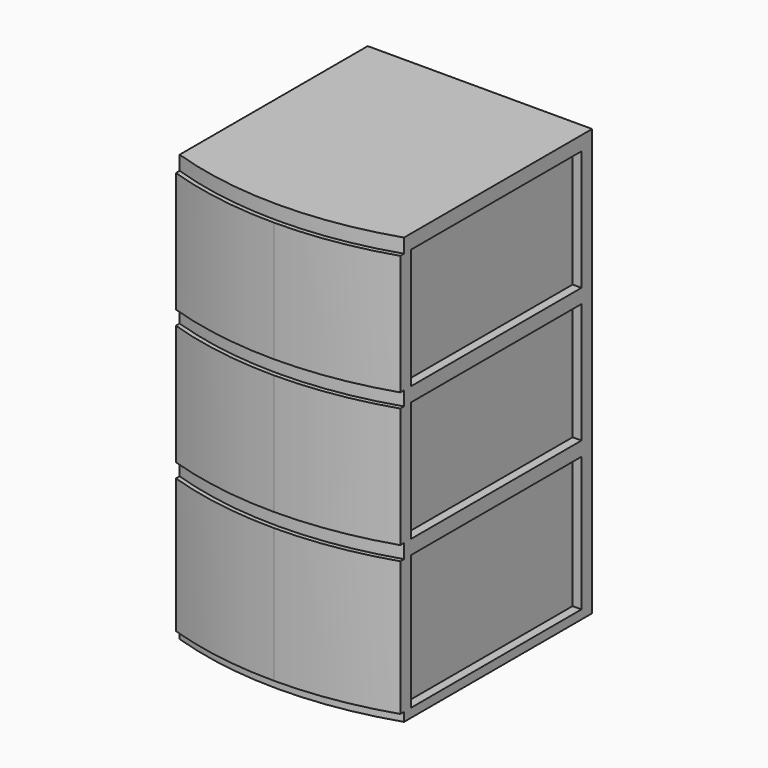
from build123d import *

# Parameters (mm, degrees)
F0_W      = 320.802
F0_H      = 609.6
F1_DEPTH  = 368.3
F3_DEPTH  = 609.601
F6_W      = 6.35
F6_H      = 20.32
F6_H_2    = 12.7
F8_W      = 304.8
F8_H      = 171.8733333333
F8_H_2    = 192.1933333333
F9_DEPTH  = 12.7
F11_DEPTH = 508


# Not quite as in the source:
# - a pattern or mirror of a feature is missing from the dataset's text; its kind, count and spacing are read off the source's solid


with BuildPart() as f1:
    # F0 (on Front) → F1 (new body)
    with BuildSketch(Plane.XZ):
        with Locations((160.401, 304.8)):
            Rectangle(F0_W, F0_H)
    extrude(amount=-F1_DEPTH)

    # F2 (on face) → F3 (cut, through all)
    with BuildSketch(Plane.XY.offset(609.6)):
        with BuildLine():
            ThreePointArc((160.401, 0), (79.2011834962, 6.3893162785), (0, 25.4))
            Line((0, 25.4), (0, 0))
            Line((0, 0), (160.401, 0))
        make_face()
        with BuildLine():
            Line((320.802, 0), (320.802, 25.4))
            ThreePointArc((320.802, 25.4), (241.6008165038, 6.3893162785), (160.401, 0))
            Line((160.401, 0), (320.802, 0))
        make_face()
    extrude(amount=-F3_DEPTH, mode=Mode.SUBTRACT)

    # F6 (on mid) → F7 (revolve, cut)
    with BuildSketch(Plane.YZ.offset(160.401)):
        with Locations((3.175, 599.44)):
            Rectangle(F6_W, F6_H)
        with Locations((3.175, 407.2466666667)):
            Rectangle(F6_W, F6_H)
        with Locations((3.175, 215.0533333333)):
            Rectangle(F6_W, F6_H)
        with Locations((3.175, 6.35)):
            Rectangle(F6_W, F6_H_2)
    revolve(axis=Axis((160.401, 519.1661575, 538.612387991), (0, 0, -1)), mode=Mode.SUBTRACT)

    # F8 (on face) → F9 (cut)
    with BuildSketch(Plane.YZ.offset(320.802)):
        with Locations((196.85, 503.3433333333)):
            Rectangle(F8_W, F8_H)
        with Locations((196.85, 311.15)):
            Rectangle(F8_W, F8_H)
        with Locations((196.85, 108.7966666667)):
            Rectangle(F8_W, F8_H_2)
    f9 = extrude(amount=-F9_DEPTH, mode=Mode.SUBTRACT)

    # F9_copies: F9 across plane
    add(f9.mirror(Plane(origin=(160.401, 0, 0), x_dir=(0, 0, -1), z_dir=(-1, 0, 0))), mode=Mode.SUBTRACT)

    # F10 (on face) → F11 (cut)
    with BuildSketch(Plane(origin=(0, 0, 0), x_dir=(1, 0, 0), z_dir=(0, 0, -1))):
        with BuildLine():
            Line((101.6, -266.7), (219.202, -266.7))
            Line((219.202, -266.7), (219.202, -112.1757760558))
            ThreePointArc((219.202, -112.1757760558), (160.401, -107.95), (101.6, -112.1757760558))
            Line((101.6, -112.1757760558), (101.6, -266.7))
        make_face()
    extrude(amount=-F11_DEPTH, mode=Mode.SUBTRACT)


solid = f1.part
